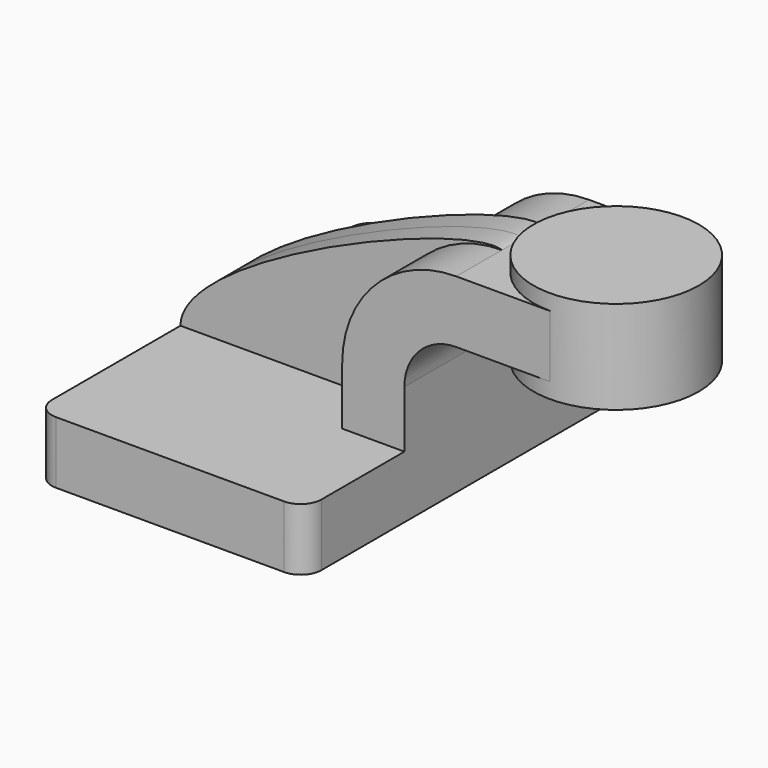
from build123d import *

# Parameters (mm, degrees)
F0_W     = 25.4762
F0_H     = 19.05
F1_DEPTH = 25.4
F2_DEPTH = 63.5
F3_DEPTH = 7.9375
F5_R     = 6.35


# Not quite as in the source:
# - a feature names something its author has since deleted; it is built from what else it names


with BuildPart() as f1:
    # F0 (on Front) → F1 (new body, symmetric)
    with BuildSketch(Plane.XZ):
        with BuildLine():
            Line((22.225, 9.525), (41.275, 9.525))
            Line((41.275, 9.525), (41.275, 27.0002))
            ThreePointArc((41.275, 27.0002), (45.9246798487, 38.2255201513), (57.15, 42.8752))
            Line((57.15, 42.8752), (60.325, 42.8752))
            Line((60.325, 42.8752), (60.325, 61.9252))
            Line((60.325, 61.9252), (57.15, 61.9252))
            ThreePointArc((57.15, 61.9252), (32.4542956671, 51.6959043329), (22.225, 27.0002))
            Line((22.225, 27.0002), (22.225, 9.525))
        make_face()
        with Locations((73.0631, 52.4002)):
            Rectangle(F0_W, F0_H)
    extrude(amount=F1_DEPTH, both=True)

    # F0 (on Front) → F2 (join, symmetric)
    with BuildSketch(Plane.XZ):
        Polygon((41.275, -9.525), (41.275, 9.525), (22.225, 9.525), (-41.275, 9.525), (-41.275, -9.525), align=None)
    extrude(amount=F2_DEPTH, both=True)

    # F0 (on Front) → F3 (join, symmetric)
    with BuildSketch(Plane.XZ):
        with BuildLine():
            Line((-41.275, 9.525), (22.225, 9.525))
            Line((22.225, 9.525), (22.225, 27.0002))
            ThreePointArc((22.225, 27.0002), (32.4542956671, 51.6959043329), (57.15, 61.9252))
            add(Edge.make_bspline(
                [(-41.275, 9.525), (-40.9908369184, 30.6630749255), (45.7423105836, 66.1747902632), (57.15, 61.9252)],
                knots=[0, 0, 0, 0, 111.5045361635, 111.5045361635, 111.5045361635, 111.5045361635], degree=3))
        make_face()
    extrude(amount=F3_DEPTH, both=True)

    # F0 (on Front) → F4 (revolve)
    with BuildSketch(Plane.XZ):
        Polygon((85.8012, 61.9252), (85.8012, 42.8752), (85.8012, 38.1), (111.125, 38.1), (111.125, 66.675), (85.8012, 66.675), align=None)
    revolve(axis=Axis((85.8012, 0, 52.3875), (0, 0, -1)))

    # F5
    f5_edges = [f1.edges().sort_by_distance(p)[0] for p in [
        (41.275, -63.5, 0),
        (-41.275, -63.5, 0),
        (41.275, 63.5, 0),
        (-41.275, 63.5, 0),
    ]]
    fillet(f5_edges, radius=F5_R)


solid = f1.part
